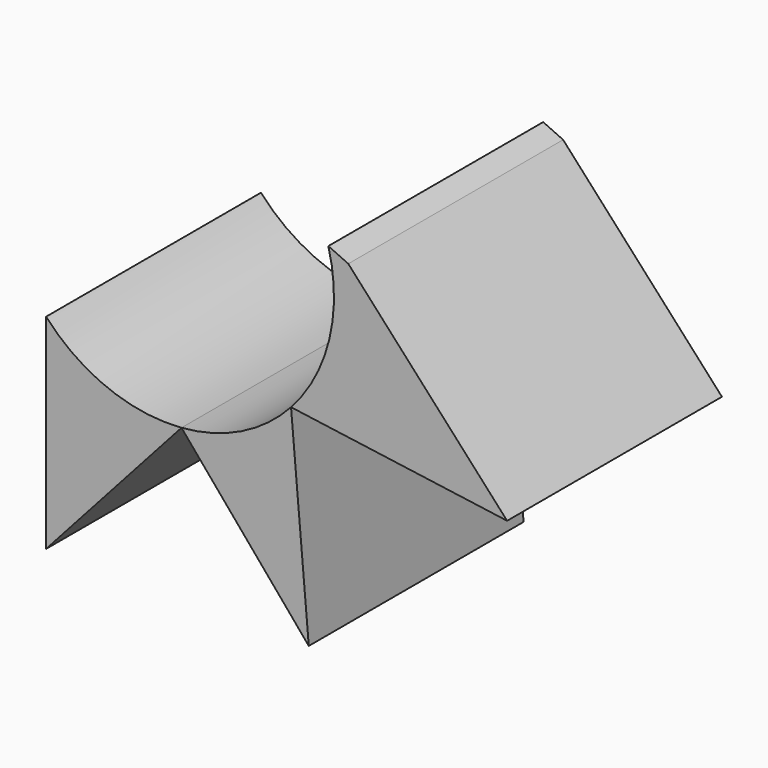
from build123d import *

# Parameters (mm, degrees)
F2_DEPTH = 25.4
F3_DEPTH = 25.4
F4_DEPTH = 25.4


# Not quite as in the source:
# - the program builds the solid bodies; features that only make, move or delete a surface that nothing else refers to are left out


with BuildPart() as f2:
    # F0 (on Front) → F2 (new body)
    with BuildSketch(Plane.XZ):
        with BuildLine():
            Line((-21.2980724055, -35.6793105602), (-8.4871734768, -21.4231418318))
            ThreePointArc((-8.4871734768, -21.4231418318), (-15.4822035317, -20.368652553), (-21.2980724055, -16.3414870052))
            Line((-21.2980724055, -16.3414870052), (-21.2980724055, -35.6793105602))
        make_face()
    extrude(amount=F2_DEPTH)


with BuildPart() as f2b:
    # F0 (on Front) → F2, piece 2 (new body)
    with BuildSketch(Plane.XZ):
        with BuildLine():
            Line((3.5508128349, -35.6793105602), (1.8730703471, -16.3414870052))
            ThreePointArc((1.8730703471, -16.3414870052), (-2.8215223771, -19.8721889655), (-8.4871734768, -21.4231418318))
            Line((-8.4871734768, -21.4231418318), (3.5508128349, -35.6793105602))
        make_face()
    extrude(amount=F2_DEPTH)


with BuildPart() as f2c:
    # F0 (on Front) → F2, piece 3 (new body)
    with BuildSketch(Plane.XZ):
        with BuildLine():
            Line((22.3111603409, -19.156107679), (7.2886282847, -2.6376740133))
            add(Edge.make_bspline(
                [(5.4032869201, -1.7767953694), (6.0356572868, -2.0719724376), (6.6644062734, -2.3594052932), (7.2886282847, -2.6376740133)],
                knots=[0.0868033089, 0.0868033089, 0.0868033089, 0.0868033089, 0.0947225706, 0.0947225706, 0.0947225706, 0.0947225706], degree=3))
            ThreePointArc((5.4032869201, -1.7767953694), (5.4951683541, -9.5092417491), (1.8730703471, -16.3414870052))
            Line((1.8730703471, -16.3414870052), (22.3111603409, -19.156107679))
        make_face()
    extrude(amount=F2_DEPTH)


with BuildPart() as f3:
    # F0 (on Front) → F3 (new body)
    with BuildSketch(Plane.XZ):
        with BuildLine():
            Line((-21.2980724055, -35.6793105602), (-8.4871734768, -21.4231418318))
            ThreePointArc((-8.4871734768, -21.4231418318), (-15.4822035317, -20.368652553), (-21.2980724055, -16.3414870052))
            Line((-21.2980724055, -16.3414870052), (-21.2980724055, -35.6793105602))
        make_face()
    extrude(amount=F3_DEPTH)


with BuildPart() as f3b:
    # F0 (on Front) → F3, piece 2 (new body)
    with BuildSketch(Plane.XZ):
        with BuildLine():
            Line((3.5508128349, -35.6793105602), (1.8730703471, -16.3414870052))
            ThreePointArc((1.8730703471, -16.3414870052), (-2.8215223771, -19.8721889655), (-8.4871734768, -21.4231418318))
            Line((-8.4871734768, -21.4231418318), (3.5508128349, -35.6793105602))
        make_face()
    extrude(amount=F3_DEPTH)


with BuildPart() as f3c:
    # F0 (on Front) → F3, piece 3 (new body)
    with BuildSketch(Plane.XZ):
        with BuildLine():
            Line((22.3111603409, -19.156107679), (7.2886282847, -2.6376740133))
            add(Edge.make_bspline(
                [(5.4032869201, -1.7767953694), (6.0356572868, -2.0719724376), (6.6644062734, -2.3594052932), (7.2886282847, -2.6376740133)],
                knots=[0.0868033089, 0.0868033089, 0.0868033089, 0.0868033089, 0.0947225706, 0.0947225706, 0.0947225706, 0.0947225706], degree=3))
            ThreePointArc((5.4032869201, -1.7767953694), (5.4951683541, -9.5092417491), (1.8730703471, -16.3414870052))
            Line((1.8730703471, -16.3414870052), (22.3111603409, -19.156107679))
        make_face()
    extrude(amount=F3_DEPTH)


with BuildPart() as f4:
    # F0 (on Front) → F4 (new body)
    with BuildSketch(Plane.XZ):
        with BuildLine():
            Line((-21.2980724055, -35.6793105602), (-8.4871734768, -21.4231418318))
            ThreePointArc((-8.4871734768, -21.4231418318), (-15.4822035317, -20.368652553), (-21.2980724055, -16.3414870052))
            Line((-21.2980724055, -16.3414870052), (-21.2980724055, -35.6793105602))
        make_face()
    extrude(amount=F4_DEPTH)


with BuildPart() as f4b:
    # F0 (on Front) → F4, piece 2 (new body)
    with BuildSketch(Plane.XZ):
        with BuildLine():
            Line((3.5508128349, -35.6793105602), (1.8730703471, -16.3414870052))
            ThreePointArc((1.8730703471, -16.3414870052), (-2.8215223771, -19.8721889655), (-8.4871734768, -21.4231418318))
            Line((-8.4871734768, -21.4231418318), (3.5508128349, -35.6793105602))
        make_face()
    extrude(amount=F4_DEPTH)


with BuildPart() as f4c:
    # F0 (on Front) → F4, piece 3 (new body)
    with BuildSketch(Plane.XZ):
        with BuildLine():
            Line((22.3111603409, -19.156107679), (7.2886282847, -2.6376740133))
            add(Edge.make_bspline(
                [(5.4032869201, -1.7767953694), (6.0356572868, -2.0719724376), (6.6644062734, -2.3594052932), (7.2886282847, -2.6376740133)],
                knots=[0.0868033089, 0.0868033089, 0.0868033089, 0.0868033089, 0.0947225706, 0.0947225706, 0.0947225706, 0.0947225706], degree=3))
            ThreePointArc((5.4032869201, -1.7767953694), (5.4951683541, -9.5092417491), (1.8730703471, -16.3414870052))
            Line((1.8730703471, -16.3414870052), (22.3111603409, -19.156107679))
        make_face()
    extrude(amount=F4_DEPTH)


solid = Compound([f2.part, f2b.part, f2c.part, f3.part, f3b.part, f3c.part, f4.part, f4b.part, f4c.part])
